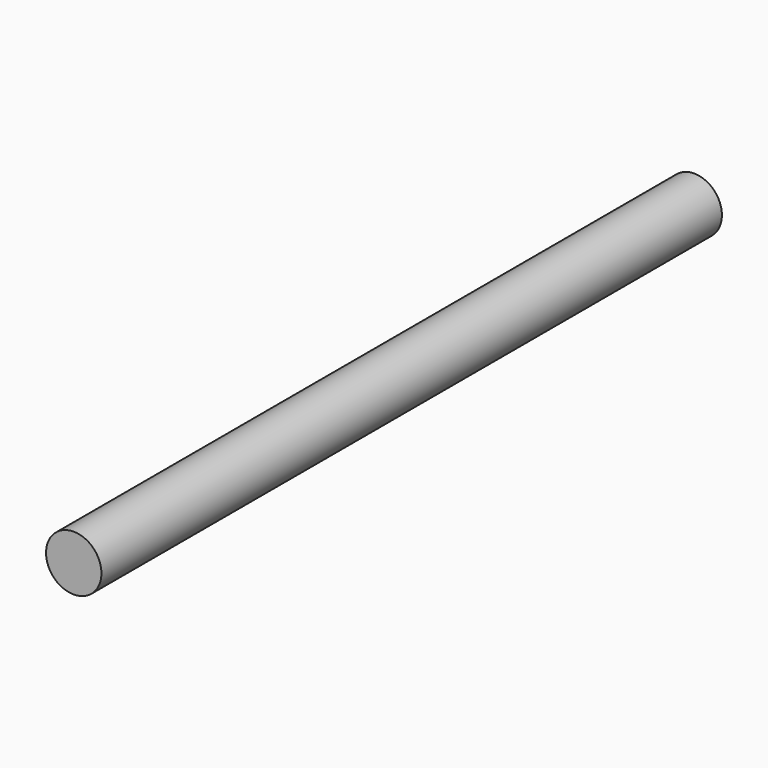
from build123d import *

# Parameters (mm, degrees)
F0_R     = 9.525
F1_DEPTH = 266.7


# Not quite as in the source:
# - the program builds the solid bodies; features that only make, move or delete a surface that nothing else refers to are left out


with BuildPart() as f1:
    # F0 (on Front) → F1 (new body)
    with BuildSketch(Plane.XZ):
        Circle(F0_R)
    extrude(amount=F1_DEPTH)


solid = f1.part
